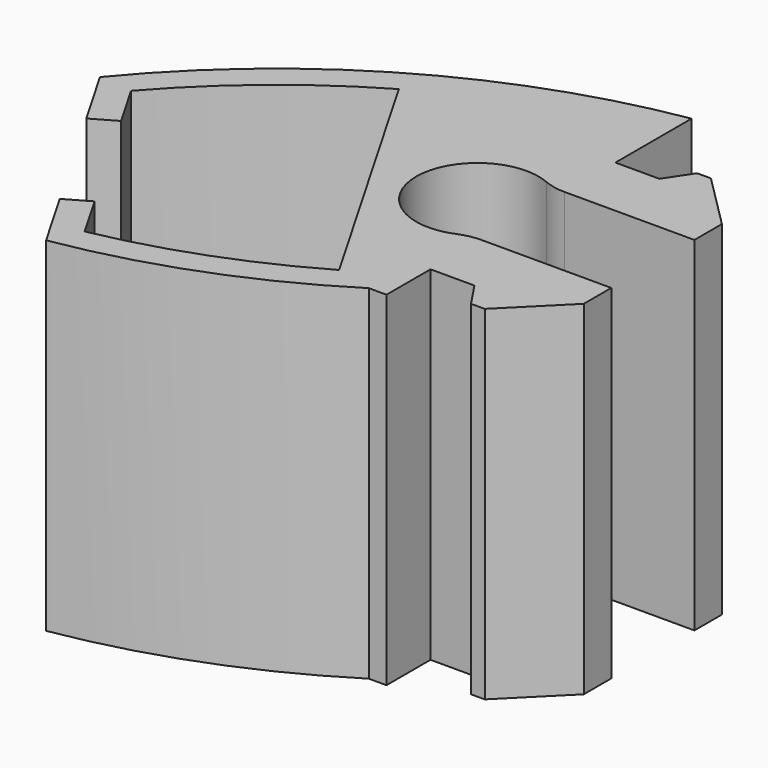
from build123d import *

# Parameters (mm, degrees)
F2_DEPTH = 10


# Not quite as in the source:
# - a feature names something its author has since deleted; it is built from what else it names


with BuildPart() as f2:
    # F1 (on Top) → F2 (new body)
    with BuildSketch(Plane.XY):
        with BuildLine():
            ThreePointArc((-20.7961524227, -0.7545254038), (-18.6080572337, 1.3728200267), (-16.1, 3.1115))
            Line((-16.1, 3.1115), (-11.6, -4.6827286341))
            ThreePointArc((-11.6, -4.6827286341), (-14.3597696428, -5.9854299259), (-17.2961524227, -6.8167032303))
            Line((-17.2961524227, -6.8167032303), (-18.0461524227, -5.5176651246))
            Line((-18.0461524227, -5.5176651246), (-18.7389727457, -5.9176651246))
            Line((-18.7389727457, -5.9176651246), (-17.7077768116, -7.703748875))
            ThreePointArc((-17.7077768116, -7.703748875), (-13.9735101965, -6.69466899), (-10.5154733964, -4.9611838136))
            Line((-10.5154733964, -4.9611838136), (-10, -4.9611838136))
            Line((-10, -4.9611838136), (-10, -3.3615))
            Line((-10, -3.3615), (-8.722, -3.3615))
            Line((-8.722, -3.3615), (-8.222, -4.1115))
            Line((-8.222, -4.1115), (-7.822, -4.1115))
            Line((-7.822, -4.1115), (-6.222, -2.5115))
            Line((-6.222, -2.5115), (-6.222, -1.5115))
            Line((-6.222, -1.5115), (-10, -1.5115))
            ThreePointArc((-10, -1.5115), (-10.319496099, -1.5437237906), (-10.6261229788, -1.6390971966))
            ThreePointArc((-10.6261229788, -1.6390971966), (-13.1042708913, 0), (-10.6261229788, 1.6390971966))
            ThreePointArc((-10.6261229788, 1.6390971966), (-10.319496099, 1.5437237906), (-10, 1.5115))
            Line((-10, 1.5115), (-6.222, 1.5115))
            Line((-6.222, 1.5115), (-6.222, 2.5115))
            Line((-6.222, 2.5115), (-7.822, 4.1115))
            Line((-7.822, 4.1115), (-8.222, 4.1115))
            Line((-8.222, 4.1115), (-8.722, 3.3615))
            Line((-8.722, 3.3615), (-10, 3.3615))
            Line((-10, 3.3615), (-10, 4.1899551795))
            Line((-10, 4.1899551795), (-10, 6.131235349))
            ThreePointArc((-10, 6.131235349), (-12.9768183038, 5.3917266036), (-15.7988859575, 4.1899551795))
            ThreePointArc((-15.7988859575, 4.1899551795), (-19.0291465574, 2.0619500516), (-21.7701686798, -0.6674797591))
            Line((-21.7701686798, -0.6674797591), (-20.7389727457, -2.4535635095))
            Line((-20.7389727457, -2.4535635095), (-20.0461524227, -2.0535635095))
            Line((-20.0461524227, -2.0535635095), (-20.7961524227, -0.7545254038))
        make_face()
    extrude(amount=F2_DEPTH)


solid = f2.part
